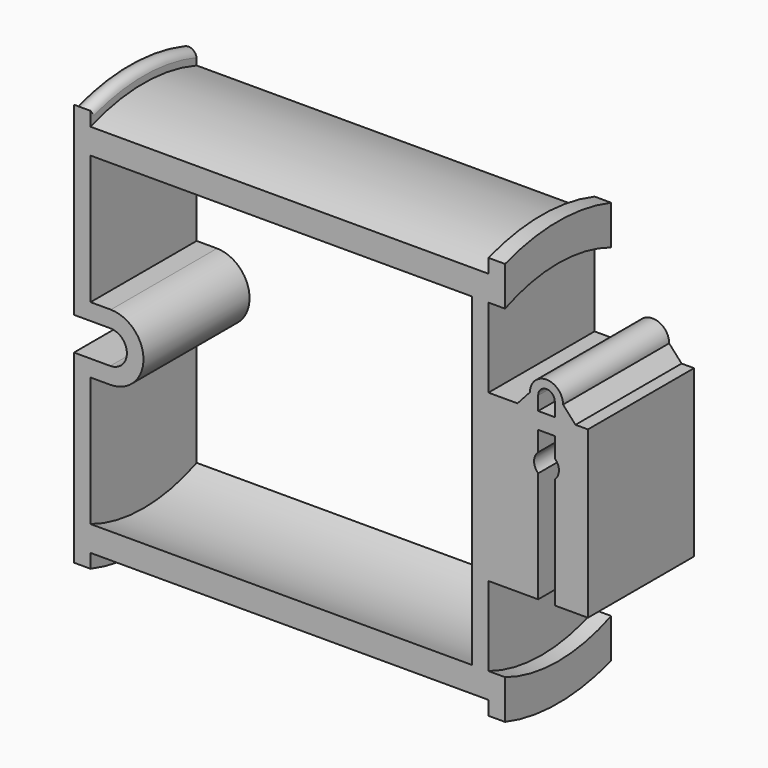
from build123d import *

# Parameters (mm, degrees)
F1_DEPTH = 25.4
F2_W     = 25.4
F2_H     = 12.7
F3_DEPTH = 3.175
F4_DEPTH = 76.2
F5_START = 76.2
F5_DEPTH = 3.175
F6_DEPTH = 3.175
F8_DEPTH = 25.4


# Not quite as in the source:
# - a feature names something its author has since deleted; it is built from what else it names


with BuildPart() as f1:
    # F0 (on Front) → F1 (new body)
    with BuildSketch(Plane.XZ):
        with BuildLine():
            Line((5.55625, 0), (0, 0))
            Line((0, 0), (0, -31.75))
            Line((0, -31.75), (9.525, -31.75))
            Line((9.525, -31.75), (9.525, -10.5061289571))
            ThreePointArc((9.525, -10.5061289571), (8.73125, -8.73125), (9.525, -6.9563710429))
            Line((9.525, -6.9563710429), (9.525, -3.175))
            Line((9.525, -3.175), (11.1125, -3.175))
            Line((11.1125, -3.175), (12.7, -3.175))
            Line((12.7, -3.175), (12.7, -6.35))
            Line((12.7, -6.35), (12.7, -6.9563710429))
            ThreePointArc((12.7, -6.9563710429), (13.49375, -8.73125), (12.7, -10.5061289571))
            Line((12.7, -10.5061289571), (12.7, -28.575))
            Line((12.7, -28.575), (12.7, -31.75))
            Line((12.7, -31.75), (19.05, -31.75))
            Line((19.05, -31.75), (19.05, 0))
            Line((19.05, 0), (16.66875, 0))
            Line((16.66875, 0), (14.2875, 2.6339585893))
            ThreePointArc((14.2875, 2.6339585893), (11.1125, 5.8089585893), (7.9375, 2.6339585893))
            Line((7.9375, 2.6339585893), (5.55625, 0))
        make_face()
        with BuildLine():
            Line((12.7, 0), (11.1125, 0))
            Line((11.1125, 0), (9.525, 0))
            Line((9.525, 0), (9.525, 2.6339585893))
            ThreePointArc((9.525, 2.6339585893), (11.1125, 4.2214585893), (12.7, 2.6339585893))
            Line((12.7, 2.6339585893), (12.7, 0))
        make_face(mode=Mode.SUBTRACT)
    extrude(amount=F1_DEPTH)

    # F2 (on face) → F3 (join)
    with BuildSketch(Plane(origin=(0, 0, 0), x_dir=(0, -1, 0), z_dir=(-1, 0, 0))):
        with BuildLine():
            ThreePointArc((0, 15.186421298), (12.7, 17.6824416941), (25.4, 15.186421298))
            Line((25.4, 15.186421298), (25.4, 20.0460244843))
            ThreePointArc((25.4, 20.0460244843), (12.7, 22.225), (0, 20.0460244843))
            Line((0, 20.0460244843), (0, 15.186421298))
        make_face()
        with BuildLine():
            Line((0, 0), (25.4, 0))
            Line((25.4, 0), (25.4, 15.186421298))
            ThreePointArc((25.4, 15.186421298), (12.7, 17.6824416941), (0, 15.186421298))
            Line((0, 15.186421298), (0, 0))
        make_face()
        with BuildLine():
            Line((0, -31.75), (0, -46.936421298))
            ThreePointArc((0, -46.936421298), (12.7, -49.4324416941), (25.4, -46.936421298))
            Line((25.4, -46.936421298), (25.4, -31.75))
            Line((25.4, -31.75), (0, -31.75))
        make_face()
        with BuildLine():
            Line((0, -46.936421298), (0, -51.7960244843))
            ThreePointArc((0, -51.7960244843), (12.7, -53.975), (25.4, -51.7960244843))
            Line((25.4, -51.7960244843), (25.4, -46.936421298))
            ThreePointArc((25.4, -46.936421298), (12.7, -49.4324416941), (0, -46.936421298))
        make_face()
        with Locations((12.7, -25.4)):
            Rectangle(F2_W, F2_H)
        with Locations((12.7, -6.35)):
            Rectangle(F2_W, F2_H)
        Polygon((0, -15.875), (0, -19.05), (25.4, -19.05), (25.4, -12.7), (0, -12.7), align=None)
    extrude(amount=F3_DEPTH)

    # F2 (on face) → F4 (join)
    with BuildSketch(Plane(origin=(0, 0, 0), x_dir=(0, -1, 0), z_dir=(-1, 0, 0))):
        with BuildLine():
            ThreePointArc((0, 15.186421298), (12.7, 17.6824416941), (25.4, 15.186421298))
            Line((25.4, 15.186421298), (25.4, 20.0460244843))
            ThreePointArc((25.4, 20.0460244843), (12.7, 22.225), (0, 20.0460244843))
            Line((0, 20.0460244843), (0, 15.186421298))
        make_face()
        with BuildLine():
            Line((0, -46.936421298), (0, -51.7960244843))
            ThreePointArc((0, -51.7960244843), (12.7, -53.975), (25.4, -51.7960244843))
            Line((25.4, -51.7960244843), (25.4, -46.936421298))
            ThreePointArc((25.4, -46.936421298), (12.7, -49.4324416941), (0, -46.936421298))
        make_face()
    extrude(amount=F4_DEPTH)

    # F2 (on face) → F5 (join)
    with BuildSketch(Plane(origin=(0, 0, 0), x_dir=(0, -1, 0), z_dir=(-1, 0, 0)).offset(F5_START)):
        with BuildLine():
            ThreePointArc((25.4, -51.7960244843), (12.7, -53.975), (0, -51.7960244843))
            Line((0, -51.7960244843), (0, -54.4783297054))
            ThreePointArc((0, -54.4783297054), (12.7, -56.5137384689), (25.4, -54.4783297054))
            Line((25.4, -54.4783297054), (25.4, -51.7960244843))
        make_face()
        with BuildLine():
            Line((0, -46.936421298), (0, -51.7960244843))
            ThreePointArc((0, -51.7960244843), (12.7, -53.975), (25.4, -51.7960244843))
            Line((25.4, -51.7960244843), (25.4, -46.936421298))
            ThreePointArc((25.4, -46.936421298), (12.7, -49.4324416941), (0, -46.936421298))
        make_face()
        with BuildLine():
            Line((0, -31.75), (0, -46.936421298))
            ThreePointArc((0, -46.936421298), (12.7, -49.4324416941), (25.4, -46.936421298))
            Line((25.4, -46.936421298), (25.4, -31.75))
            Line((25.4, -31.75), (0, -31.75))
        make_face()
        with Locations((12.7, -25.4)):
            Rectangle(F2_W, F2_H)
        with Locations((12.7, -6.35)):
            Rectangle(F2_W, F2_H)
        with BuildLine():
            Line((0, 0), (25.4, 0))
            Line((25.4, 0), (25.4, 15.186421298))
            ThreePointArc((25.4, 15.186421298), (12.7, 17.6824416941), (0, 15.186421298))
            Line((0, 15.186421298), (0, 0))
        make_face()
        with BuildLine():
            ThreePointArc((0, 15.186421298), (12.7, 17.6824416941), (25.4, 15.186421298))
            Line((25.4, 15.186421298), (25.4, 20.0460244843))
            ThreePointArc((25.4, 20.0460244843), (12.7, 22.225), (0, 20.0460244843))
            Line((0, 20.0460244843), (0, 15.186421298))
        make_face()
        with BuildLine():
            ThreePointArc((0, 20.0460244843), (12.7, 22.225), (25.4, 20.0460244843))
            Line((25.4, 20.0460244843), (25.4, 22.7283297054))
            ThreePointArc((25.4, 22.7283297054), (12.7, 24.7637384689), (0, 22.7283297054))
            Line((0, 22.7283297054), (0, 20.0460244843))
        make_face()
    extrude(amount=F5_DEPTH)

    # F2 (on face) → F6 (join)
    with BuildSketch(Plane(origin=(0, 0, 0), x_dir=(0, -1, 0), z_dir=(-1, 0, 0))):
        with BuildLine():
            ThreePointArc((0, 20.0460244843), (12.7, 22.225), (25.4, 20.0460244843))
            Line((25.4, 20.0460244843), (25.4, 22.7283297054))
            ThreePointArc((25.4, 22.7283297054), (12.7, 24.7637384689), (0, 22.7283297054))
            Line((0, 22.7283297054), (0, 20.0460244843))
        make_face()
        with BuildLine():
            ThreePointArc((0, 15.186421298), (12.7, 17.6824416941), (25.4, 15.186421298))
            Line((25.4, 15.186421298), (25.4, 20.0460244843))
            ThreePointArc((25.4, 20.0460244843), (12.7, 22.225), (0, 20.0460244843))
            Line((0, 20.0460244843), (0, 15.186421298))
        make_face()
        with BuildLine():
            Line((0, -46.936421298), (0, -51.7960244843))
            ThreePointArc((0, -51.7960244843), (12.7, -53.975), (25.4, -51.7960244843))
            Line((25.4, -51.7960244843), (25.4, -46.936421298))
            ThreePointArc((25.4, -46.936421298), (12.7, -49.4324416941), (0, -46.936421298))
        make_face()
        with BuildLine():
            ThreePointArc((25.4, -51.7960244843), (12.7, -53.975), (0, -51.7960244843))
            Line((0, -51.7960244843), (0, -54.4783297054))
            ThreePointArc((0, -54.4783297054), (12.7, -56.5137384689), (25.4, -54.4783297054))
            Line((25.4, -54.4783297054), (25.4, -51.7960244843))
        make_face()
    extrude(amount=-F6_DEPTH)

    # F7 (on face) → F8 (join)
    with BuildSketch(Plane(origin=(0, 0, 0), x_dir=(-1, 0, 0), z_dir=(0, 1, 0))):
        with BuildLine():
            ThreePointArc((72.300083342, -12.7020545776), (72.4126137623, -12.7000004406), (72.5251462844, -12.7019360086))
            Line((72.5251462844, -12.7019360086), (76.2, -12.7))
            Line((76.2, -12.7), (76.2, -9.5260270395))
            Line((76.2, -9.5260270395), (72.5284895273, -9.5260270395))
            Line((72.5284895273, -9.5260270395), (72.300083342, -9.5260270395))
            ThreePointArc((72.300083342, -9.5260270395), (66.0645431997, -15.9321038554), (72.4142864347, -22.225))
            Line((72.4142864347, -22.225), (76.2, -22.225))
            Line((76.2, -22.225), (76.2, -19.05))
            Line((76.2, -19.05), (72.4142864347, -19.05))
            ThreePointArc((72.4142864347, -19.05), (69.2398001206, -15.9321107863), (72.300083342, -12.7020545776))
        make_face()
    extrude(amount=-F8_DEPTH)

    # F9: sweep along a path in F9_path
    with BuildLine(Plane(origin=(-79.375, 0, 22.7283297054), x_dir=(0, 0, -1), z_dir=(-1, 0, 0))) as f9_path:
        ThreePointArc((0, 0), (-2.0354087635, 12.7), (0, 25.4))
    # F7 (on face) → F9 (sweep, cut)
    with BuildSketch(Plane(origin=(0, 0, 0), x_dir=(-1, 0, 0), z_dir=(0, 1, 0))):
        with BuildLine():
            ThreePointArc((76.2, 21.3871770949), (77.7875, 22.7182272858), (79.375, 21.3871770949))
            Line((79.375, 21.3871770949), (79.375, 22.7283297054))
            Line((79.375, 22.7283297054), (77.7875, 22.7283297054))
            Line((77.7875, 22.7283297054), (76.2, 22.7283297054))
            Line((76.2, 22.7283297054), (76.2, 21.3871770949))
        make_face()
    sweep(path=f9_path.line, mode=Mode.SUBTRACT)


solid = f1.part
